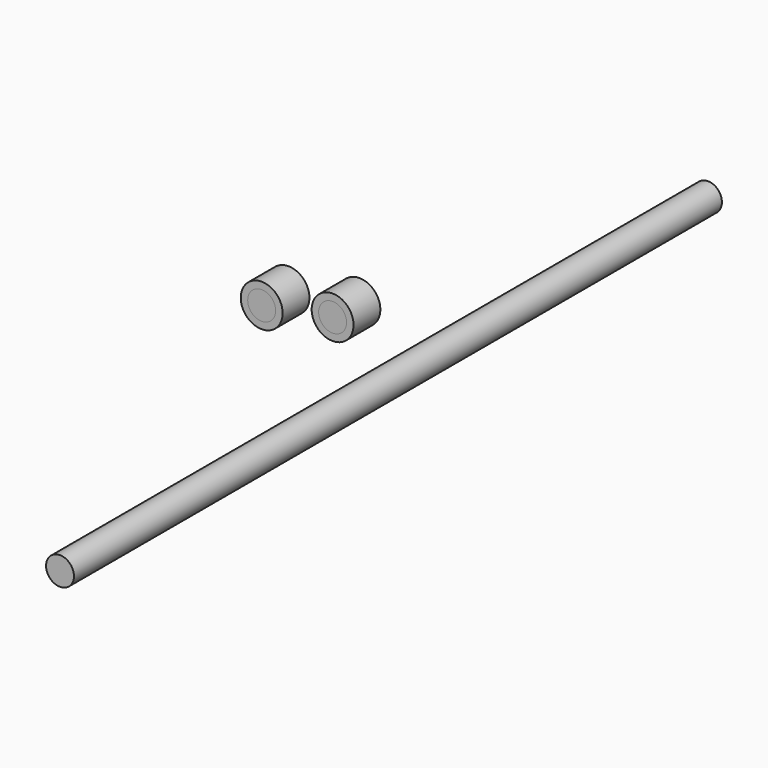
from build123d import *

# Parameters (mm, degrees)
F0_R     = 6.35
F1_DEPTH = 184.15
F0_R_2   = 9.525
F2_DEPTH = 7.62
F3_DEPTH = 7.62


with BuildPart() as f1:
    # F0 (on Front) → F1 (new body, symmetric)
    with BuildSketch(Plane.XZ):
        Circle(F0_R)
    extrude(amount=F1_DEPTH, both=True)


with BuildPart() as f2:
    # F0 (on Front) → F2 (new body, symmetric)
    with BuildSketch(Plane.XZ):
        with Locations((-49.524263, 18.436041)):
            Circle(F0_R_2)
        with BuildLine():
            ThreePointArc((-49.524263, 24.786041), (-45.034134, 22.926169), (-43.174263, 18.436041))
            ThreePointArc((-43.174263, 18.436041), (-45.034134, 13.945913), (-49.524263, 12.086041))
            ThreePointArc((-49.524263, 12.086041), (-55.874263, 18.436041), (-49.524263, 24.786041))
        make_face(mode=Mode.SUBTRACT)
    extrude(amount=F2_DEPTH, both=True)


with BuildPart() as f2b:
    # F0 (on Front) → F2, piece 2 (new body, symmetric)
    with BuildSketch(Plane.XZ):
        with Locations((-17.272001, 24.194907)):
            Circle(F0_R_2)
        with BuildLine():
            ThreePointArc((-17.272001, 30.544907), (-12.781873, 28.685035), (-10.922001, 24.194907))
            ThreePointArc((-10.922001, 24.194907), (-12.781873, 19.704779), (-17.272001, 17.844907))
            ThreePointArc((-17.272001, 17.844907), (-23.622001, 24.194907), (-17.272001, 30.544907))
        make_face(mode=Mode.SUBTRACT)
    extrude(amount=F2_DEPTH, both=True)


with BuildPart() as f3:
    # F0 (on Front) → F3 (new body)
    with BuildSketch(Plane.XZ):
        with BuildLine():
            Line((-17.272001, 17.844907), (-17.272001, 30.544907))
            ThreePointArc((-17.272001, 30.544907), (-23.622001, 24.194907), (-17.272001, 17.844907))
        make_face()
        with BuildLine():
            ThreePointArc((-17.272001, 17.844907), (-12.781873, 19.704779), (-10.922001, 24.194907))
            ThreePointArc((-10.922001, 24.194907), (-12.781873, 28.685035), (-17.272001, 30.544907))
            Line((-17.272001, 30.544907), (-17.272001, 17.844907))
        make_face()
    extrude(amount=F3_DEPTH)


with BuildPart() as f3b:
    # F0 (on Front) → F3, piece 2 (new body)
    with BuildSketch(Plane.XZ):
        with BuildLine():
            Line((-49.524263, 12.086041), (-49.524263, 24.786041))
            ThreePointArc((-49.524263, 24.786041), (-55.874263, 18.436041), (-49.524263, 12.086041))
        make_face()
        with BuildLine():
            ThreePointArc((-49.524263, 12.086041), (-45.034134, 13.945913), (-43.174263, 18.436041))
            ThreePointArc((-43.174263, 18.436041), (-45.034134, 22.926169), (-49.524263, 24.786041))
            Line((-49.524263, 24.786041), (-49.524263, 12.086041))
        make_face()
    extrude(amount=F3_DEPTH)


solid = Compound([f1.part, f2.part, f2b.part, f3.part, f3b.part])
